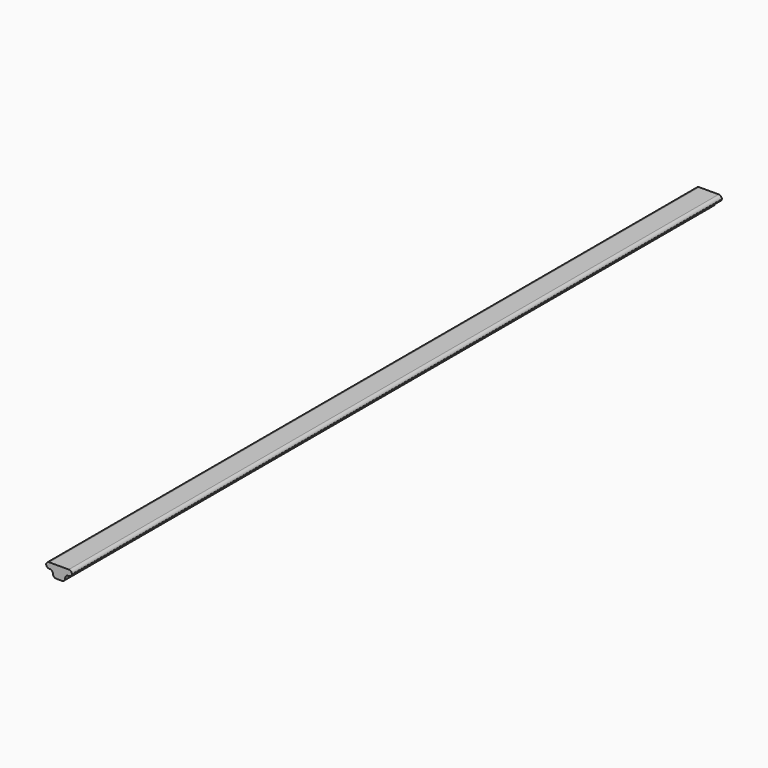
from build123d import *

# Parameters (mm, degrees)
F1_DEPTH    = 500.5
F2_T1_DEPTH = 500.5
F2_T3_DEPTH = 510.5


# Not quite as in the source:
# - a fillet or chamfer that OpenCascade refuses, or shapes differently, is made with other operations: its cross-section is extruded or revolved along the edge and cut away or added


with BuildPart() as f1:
    # F0 (on Front) → F1 (new body)
    with BuildSketch(Plane.XZ):
        Polygon((8, 0), (0, 0), (-8, 0), (-8, -3.5), (-3.75, -3.5), (-3.75, -7.5), (3.75, -7.5), (3.75, -3.5), (8, -3.5), align=None)
    extrude(amount=F1_DEPTH)

    # F2: fillet of radius 2 on 8 edges, made by hand

    # F2_s2 → F2_t1 (join)
    with BuildSketch(Plane.XZ):
        with BuildLine():
            ThreePointArc((5.75, -3.5), (4.3357864376, -4.0857864376), (3.75, -5.5))
            Line((3.75, -5.5), (3.75, -3.5))
            Line((3.75, -3.5), (5.75, -3.5))
        make_face()
        with BuildLine():
            ThreePointArc((-3.75, -5.5), (-4.3357864376, -4.0857864376), (-5.75, -3.5))
            Line((-5.75, -3.5), (-3.75, -3.5))
            Line((-3.75, -3.5), (-3.75, -5.5))
        make_face()
    extrude(amount=F2_T1_DEPTH)

    # F2_s4 → F2_t3 (cut)
    with BuildSketch(Plane.XZ.offset(-5)):
        with BuildLine():
            ThreePointArc((1.75, -7.5), (3.1642135624, -6.9142135624), (3.75, -5.5))
            Line((3.75, -5.5), (3.75, -7.5))
            Line((3.75, -7.5), (1.75, -7.5))
        make_face()
        with BuildLine():
            ThreePointArc((-3.75, -5.5), (-3.1642135624, -6.9142135624), (-1.75, -7.5))
            Line((-1.75, -7.5), (-3.75, -7.5))
            Line((-3.75, -7.5), (-3.75, -5.5))
        make_face()
        with BuildLine():
            ThreePointArc((-8, -1.5), (-7.4142135624, -2.9142135624), (-6, -3.5))
            Line((-6, -3.5), (-8, -3.5))
            Line((-8, -3.5), (-8, -1.5))
        make_face()
        with BuildLine():
            ThreePointArc((-6, 0), (-7.4142135624, -0.5857864376), (-8, -2))
            Line((-8, -2), (-8, 0))
            Line((-8, 0), (-6, 0))
        make_face()
        with BuildLine():
            ThreePointArc((8, -1.5), (7.4142135624, -2.9142135624), (6, -3.5))
            Line((6, -3.5), (8, -3.5))
            Line((8, -3.5), (8, -1.5))
        make_face()
        with BuildLine():
            ThreePointArc((6, 0), (7.4142135624, -0.5857864376), (8, -2))
            Line((8, -2), (8, 0))
            Line((8, 0), (6, 0))
        make_face()
    extrude(amount=F2_T3_DEPTH, mode=Mode.SUBTRACT)


solid = f1.part
